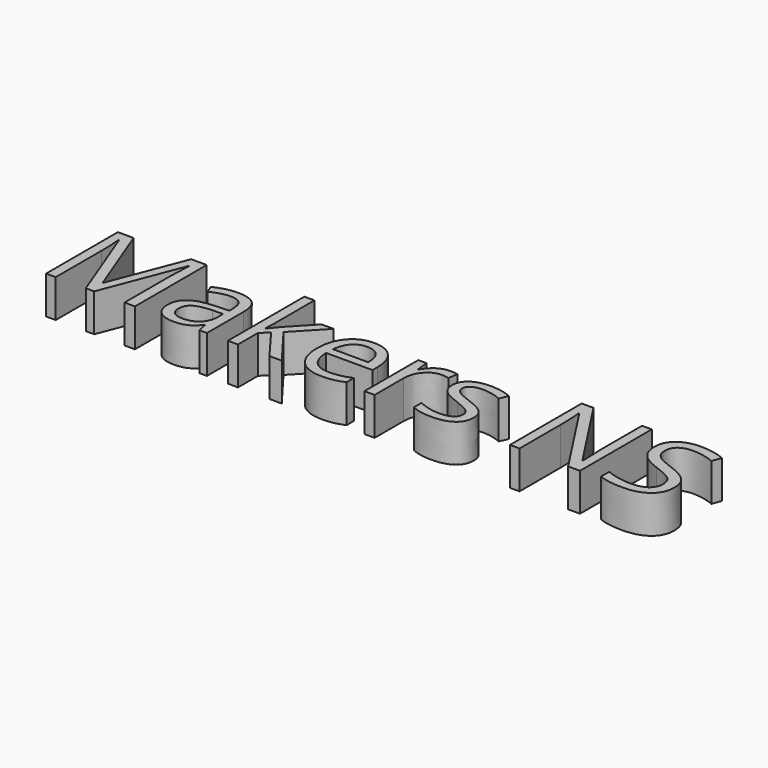
from build123d import *

# Parameters (mm, degrees)
F0_TEXT_SIZE = 42.2251850574
F1_DEPTH     = 12.7


# Not quite as in the source:
# - Text() gives the source's letters only with a copy of the font that has no kerning and outlines rounded to 1/6400 em; it was checked with that copy


with BuildPart() as f1:
    # F0 (on Top) → F1 (new body)
    with BuildSketch(Plane.XY):
        with Locations((-44.4772295216, -30.4021332413)):
            Text('Makers NS', F0_TEXT_SIZE, font='Open Sans', text_align=(TextAlign.LEFT, TextAlign.BOTTOM))
    extrude(amount=F1_DEPTH)


solid = f1.part
